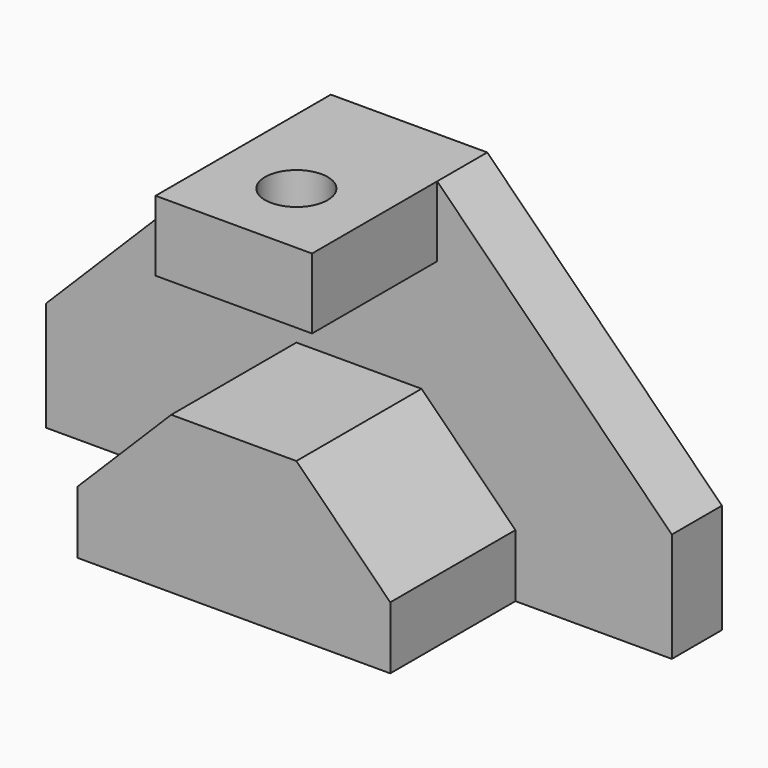
from build123d import *

# Parameters (mm, degrees)
F1_DEPTH = 12.7
F3_W     = 25.4
F3_H     = 31.75
F5_DEPTH = 31.75
F6_W     = 31.75
F6_H     = 14.2875
F7_DEPTH = 31.75
F8_R     = 6.35
F9_DEPTH = 14.3002


# Not quite as in the source:
# - a feature names something its author has since deleted; it is built from what else it names


with BuildPart() as f1:
    # F0 (on Front) → F1 (new body)
    with BuildSketch(Plane.XZ):
        Polygon((16.4174322337, 52.9738886915), (-15.3325677663, 52.9738886915), (-62.9575677663, 5.3488886915), (-62.9575677663, -16.8761113085), (64.0424322337, -16.8761113085), (64.0424322337, 5.3488886915), align=None)
    extrude(amount=F1_DEPTH)

    # F4 (on face) + F2 (on face) + F3 (on face) → F5 (join)
    with BuildSketch(Plane.XZ.offset(12.7)):
        Polygon((-31.2075677663, -4.1761113085), (-31.2075677663, -16.8761113085), (-12.1575677663, -16.8761113085), (-12.1575677663, 14.8738886915), align=None)
    with BuildSketch(Plane.XZ.offset(12.7)):
        Polygon((32.2924322337, -4.1761113085), (13.2424322337, 14.8738886915), (13.2424322337, -16.8761113085), (32.2924322337, -16.8761113085), align=None)
    with BuildSketch(Plane.XZ.offset(12.7)):
        with Locations((0.5424322337, -1.0011113085)):
            Rectangle(F3_W, F3_H)
    extrude(amount=F5_DEPTH)

    # F6 (on face) → F7 (join)
    with BuildSketch(Plane.XZ.offset(12.7)):
        with Locations((0.5424322337, 45.8301386915)):
            Rectangle(F6_W, F6_H)
    extrude(amount=F7_DEPTH)

    # F8 (on face) → F9 (cut)
    with BuildSketch(Plane.XY.offset(52.9738886915)):
        with Locations((0.5424322337, -28.575)):
            Circle(F8_R)
    extrude(amount=-F9_DEPTH, mode=Mode.SUBTRACT)


solid = f1.part
